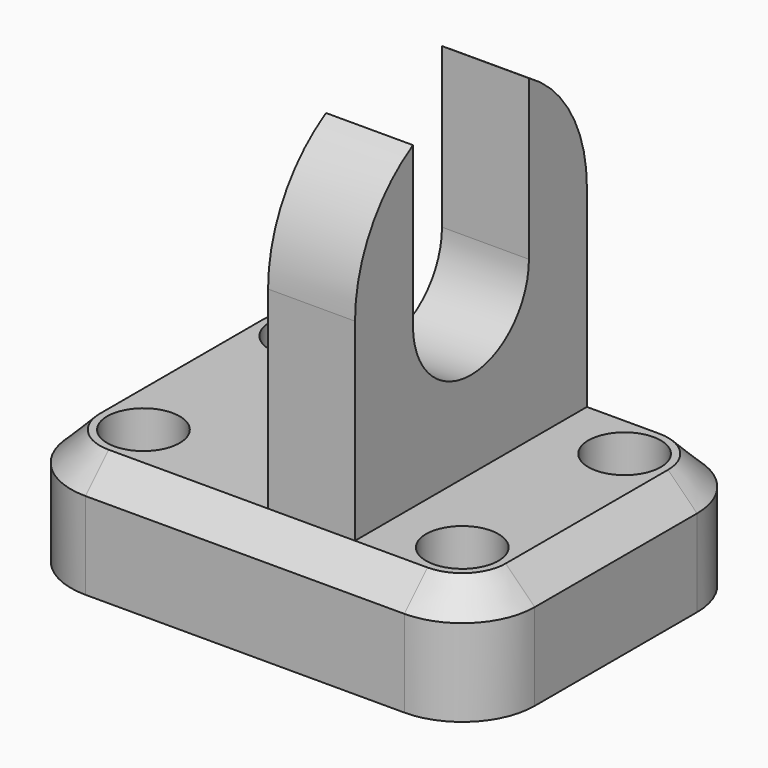
from build123d import *

# Parameters (mm, degrees)
F0_W         = 101.6
F0_H         = 76.2
F1_DEPTH     = 25.4
F2_R         = 15.875
F3_R         = 15.875
F4_R         = 15.875
F5_R         = 15.875
F7_D         = 15.875
F8_SIZE      = 6.35
F9_W         = 19.05
F9_H         = 63.5
F10_DEPTH    = 69.85
F12_DEPTH    = 25.4
F13_T1_DEPTH = 156.5315328508
F14_T1_DEPTH = 156.5315328508


# Not quite as in the source:
# - a fillet or chamfer that OpenCascade refuses, or shapes differently, is made with other operations: its cross-section is extruded or revolved along the edge and cut away or added


with BuildPart() as f1:
    # F0 (on Top) → F1 (new body)
    with BuildSketch(Plane.XY):
        with Locations((6.2353381336, -17.6054243982)):
            Rectangle(F0_W, F0_H)
    extrude(amount=F1_DEPTH)

    # F2
    f2_edges = [f1.edges().sort_by_distance(p)[0] for p in [
        (57.035338, -55.705424, 12.7),
    ]]
    fillet(f2_edges, radius=F2_R)

    # F3
    f3_edges = [f1.edges().sort_by_distance(p)[0] for p in [
        (-44.564662, -55.705424, 12.7),
    ]]
    fillet(f3_edges, radius=F3_R)

    # F4
    f4_edges = [f1.edges().sort_by_distance(p)[0] for p in [
        (-44.564662, 20.494576, 12.7),
    ]]
    fillet(f4_edges, radius=F4_R)

    # F5
    f5_edges = [f1.edges().sort_by_distance(p)[0] for p in [
        (57.035338, 20.494576, 12.7),
    ]]
    fillet(f5_edges, radius=F5_R)

    # F7 (through all)
    with Locations(Plane(origin=(0, 0, 0), x_dir=(1, 0, 0), z_dir=(0, 0, -1))):
        with Locations((-28.6896618664, 39.8304243982), (41.1603381336, 39.8304243982), (41.1603381336, -4.6195756018), (-28.6896618664, -4.6195756018)):
            Hole(F7_D / 2)

    # F8
    f8_edges = [f1.edges().sort_by_distance(p)[0] for p in [
        (6.235338, -55.705424, 25.4),
        (6.235338, 20.494576, 25.4),
        (52.385658, 15.844896, 25.4),
        (-39.914982, 15.844896, 25.4),
        (57.035338, -17.605424, 25.4),
        (-44.564662, -17.605424, 25.4),
        (52.385658, -51.055745, 25.4),
        (-39.914982, -51.055745, 25.4),
    ]]
    chamfer(f8_edges, length=F8_SIZE)

    # F9 (on face) → F10 (join)
    with BuildSketch(Plane.XY.offset(25.4)):
        with Locations((15.7603381336, -17.6054243982)):
            Rectangle(F9_W, F9_H)
    extrude(amount=F10_DEPTH)

    # F11 (on face) → F12 (cut)
    with BuildSketch(Plane(origin=(6.2353381336, 0, 0), x_dir=(0, -1, 0), z_dir=(-1, 0, 0))):
        with BuildLine():
            ThreePointArc((1.7304243982, 60.325), (17.6054243982, 44.45), (33.4804243982, 60.325))
            ThreePointArc((33.4804243982, 60.325), (17.6054243982, 76.2), (1.7304243982, 60.325))
        make_face()
        with BuildLine():
            ThreePointArc((1.7304243982, 60.325), (17.6054243982, 76.2), (33.4804243982, 60.325))
            Line((33.4804243982, 60.325), (33.4804243982, 95.25))
            Line((33.4804243982, 95.25), (1.7304243982, 95.25))
            Line((1.7304243982, 95.25), (1.7304243982, 60.325))
        make_face()
    extrude(amount=-F12_DEPTH, mode=Mode.SUBTRACT)

    # F13: fillet of radius 31.75 on 1 edges, made by hand

    # F13_s2 → F13_t1 (cut)
    with BuildSketch(Plane.YZ.offset(-62.5054282918)):
        with BuildLine():
            ThreePointArc((-33.4804243982, 95.25), (-45.1017309683, 83.6286934298), (-49.3554243982, 67.7536934298))
            Line((-49.3554243982, 67.7536934298), (-49.3554243982, 95.25))
            Line((-49.3554243982, 95.25), (-33.4804243982, 95.25))
        make_face()
    extrude(amount=F13_T1_DEPTH, mode=Mode.SUBTRACT)

    # F14: fillet of radius 31.75 on 1 edges, made by hand

    # F14_s2 → F14_t1 (cut)
    with BuildSketch(Plane.YZ.offset(-62.5054282918)):
        with BuildLine():
            ThreePointArc((14.1445756018, 67.7536934298), (9.890882172, 83.6286934298), (-1.7304243982, 95.25))
            Line((-1.7304243982, 95.25), (14.1445756018, 95.25))
            Line((14.1445756018, 95.25), (14.1445756018, 67.7536934298))
        make_face()
    extrude(amount=F14_T1_DEPTH, mode=Mode.SUBTRACT)


solid = f1.part
